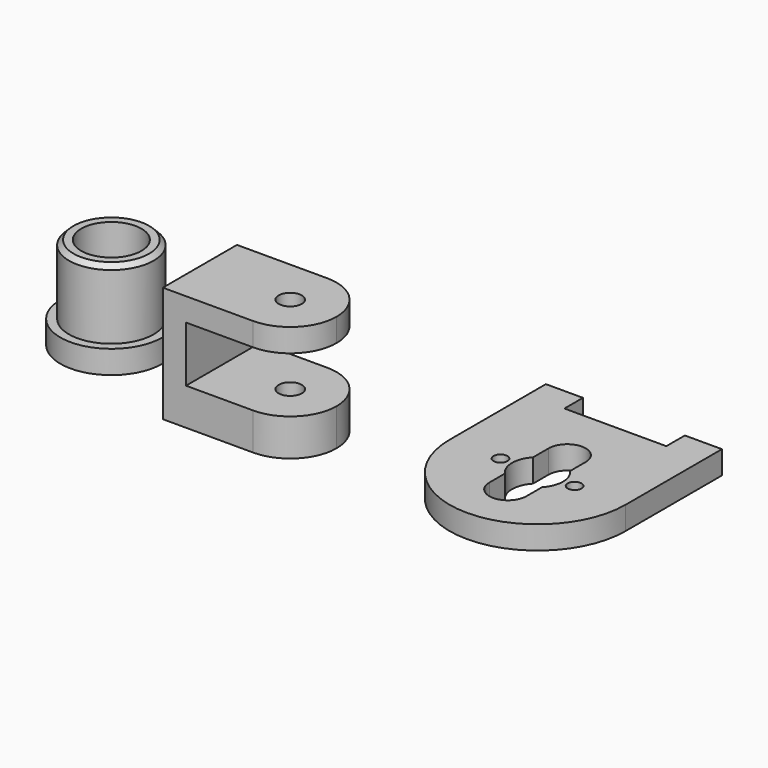
from build123d import *

# Parameters (mm, degrees)
F0_R      = 9.15
F0_R_2    = 6.5
F1_DEPTH  = 20
F0_R_3    = 11
F2_DEPTH  = 5
F3_SIZE   = 1
F5_DEPTH  = 10
F6_R      = 9.99999
F7_R      = 2.5
F8_DEPTH  = 25.001
F9_R      = 1.5
F10_DEPTH = 5


# Not quite as in the source:
# - a fillet or chamfer is up to 0.001 mm smaller than in the source, because OpenCascade refuses the exact size


with BuildPart() as f1:
    # F0 (on Top) → F1 (new body)
    with BuildSketch(Plane.XY):
        Circle(F0_R)
        Circle(F0_R_2, mode=Mode.SUBTRACT)
    extrude(amount=F1_DEPTH)

    # F0 (on Top) → F2 (join)
    with BuildSketch(Plane.XY):
        Circle(F0_R_3)
        Circle(F0_R, mode=Mode.SUBTRACT)
    extrude(amount=F2_DEPTH)

    # F3
    f3_edges = [f1.edges().sort_by_distance(p)[0] for p in [
        (-9.15, 0, 20),
    ]]
    chamfer(f3_edges, length=F3_SIZE)


with BuildPart() as f5:
    # F4 (on Front) → F5 (new body, symmetric)
    with BuildSketch(Plane.XZ):
        Polygon((48.6184198422, 16.1811771655), (48.6184198422, 21.1811771655), (19.1184198422, 21.1811771655), (19.1184198422, -3.8188228345), (48.6184198422, -3.8188228345), (48.6184198422, 4.1811771655), (24.1184198422, 4.1811771655), (24.1184198422, 16.1811771655), align=None)
    extrude(amount=F5_DEPTH, both=True)

    # F6 (radius 10 in the source; OpenCascade refuses exactly that, so slightly less here)
    f6_edges = [f5.edges().sort_by_distance(p)[0] for p in [
        (48.61842, -10, 18.681177),
        (48.61842, 10, 18.681177),
        (48.61842, 10, 0.181177),
        (48.61842, -10, 0.181177),
    ]]
    fillet(f6_edges, radius=F6_R)

    # F7 (on face) → F8 (cut, through all)
    with BuildSketch(Plane.XY.offset(21.1811771655)):
        with Locations((38.6184198422, 0)):
            Circle(F7_R)
    extrude(amount=-F8_DEPTH, mode=Mode.SUBTRACT)


with BuildPart() as f10:
    # F9 (on Top) → F10 (new body)
    with BuildSketch(Plane.XY):
        with BuildLine():
            Line((72.1199496662, 27.1096767731), (72.1199496662, 1.1096767731))
            ThreePointArc((72.1199496662, 1.1096767731), (91.1199496662, -17.8903232269), (110.1199496662, 1.1096767731))
            Line((110.1199496662, 1.1096767731), (110.1199496662, 27.1096767731))
            Line((110.1199496662, 27.1096767731), (102.1199496662, 27.1096767731))
            Line((102.1199496662, 27.1096767731), (102.1199496662, 22.1096767731))
            Line((102.1199496662, 22.1096767731), (80.1199496662, 22.1096767731))
            Line((80.1199496662, 22.1096767731), (80.1199496662, 27.1096767731))
            Line((80.1199496662, 27.1096767731), (72.1199496662, 27.1096767731))
        make_face()
        with Locations((83.1199496662, 1.1096767731)):
            Circle(F9_R, mode=Mode.SUBTRACT)
        with BuildLine():
            ThreePointArc((87.1199496662, -2.6652404445), (85.6199496662, 1.1096767731), (87.1199496662, 4.8845939907))
            Line((87.1199496662, 4.8845939907), (87.1199496662, 9.1096767731))
            ThreePointArc((87.1199496662, 9.1096767731), (91.1199496662, 13.1096767731), (95.1199496662, 9.1096767731))
            Line((95.1199496662, 9.1096767731), (95.1199496662, 4.8845939907))
            ThreePointArc((95.1199496662, 4.8845939907), (96.6199496662, 1.1096767731), (95.1199496662, -2.6652404445))
            Line((95.1199496662, -2.6652404445), (95.1199496662, -6.8903232269))
            ThreePointArc((95.1199496662, -6.8903232269), (91.1199496662, -10.8903232269), (87.1199496662, -6.8903232269))
            Line((87.1199496662, -6.8903232269), (87.1199496662, -2.6652404445))
        make_face(mode=Mode.SUBTRACT)
        with Locations((99.1199496662, 1.1096767731)):
            Circle(F9_R, mode=Mode.SUBTRACT)
    extrude(amount=F10_DEPTH)


solid = Compound([f1.part, f5.part, f10.part])
